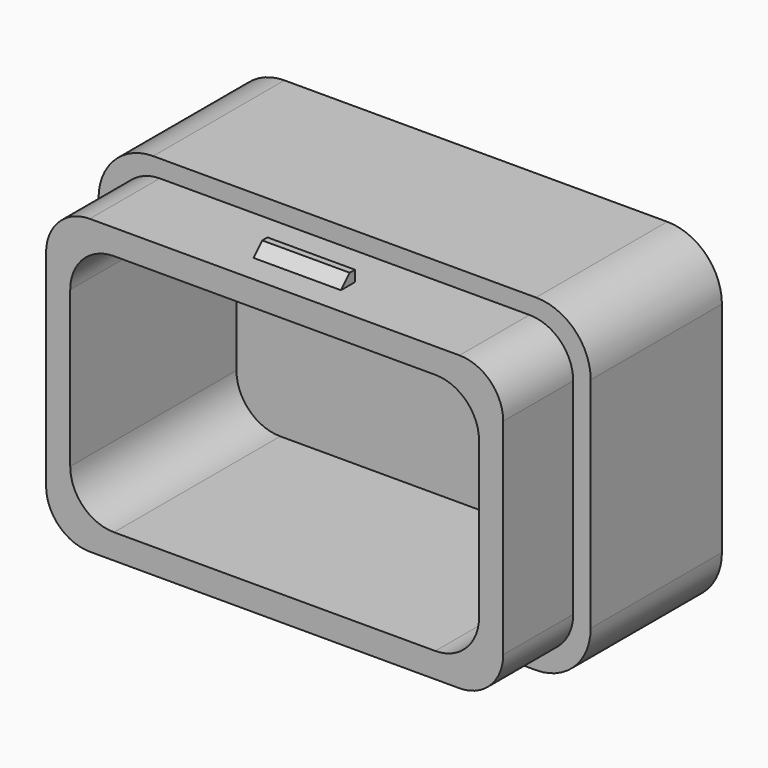
from build123d import *

# Parameters (mm, degrees)
F1_DEPTH = 19.05
F2_DEPTH = 29.21
F3_DEPTH = 5.08
F4_W     = 10.16
F4_H     = 2.032
F5_DEPTH = 1.27
F6_SIZE  = 1.26999


# Not quite as in the source:
# - a fillet or chamfer is up to 0.001 mm smaller than in the source, because OpenCascade refuses the exact size


with BuildPart() as f1:
    # F0 (on Front) → F1 (new body)
    with BuildSketch(Plane.XZ):
        with BuildLine():
            ThreePointArc((28.575, 12.7), (26.7151280605, 17.1901280605), (22.225, 19.05))
            Line((22.225, 19.05), (-22.225, 19.05))
            ThreePointArc((-22.225, 19.05), (-26.7151280605, 17.1901280605), (-28.575, 12.7))
            Line((-28.575, 12.7), (-28.575, -12.7))
            ThreePointArc((-28.575, -12.7), (-26.7151280605, -17.1901280605), (-22.225, -19.05))
            Line((-22.225, -19.05), (22.225, -19.05))
            ThreePointArc((22.225, -19.05), (26.7151280605, -17.1901280605), (28.575, -12.7))
            Line((28.575, -12.7), (28.575, 12.7))
        make_face()
        with BuildLine():
            Line((-21.463, 17.018), (21.463, 17.018))
            ThreePointArc((21.463, 17.018), (25.0551024484, 15.5301024484), (26.543, 11.938))
            Line((26.543, 11.938), (26.543, -11.938))
            ThreePointArc((26.543, -11.938), (25.0551024484, -15.5301024484), (21.463, -17.018))
            Line((21.463, -17.018), (-21.463, -17.018))
            ThreePointArc((-21.463, -17.018), (-25.0551024484, -15.5301024484), (-26.543, -11.938))
            Line((-26.543, -11.938), (-26.543, 11.938))
            ThreePointArc((-26.543, 11.938), (-25.0551024484, 15.5301024484), (-21.463, 17.018))
        make_face(mode=Mode.SUBTRACT)
    extrude(amount=F1_DEPTH)

    # F0 (on Front) → F2 (join)
    with BuildSketch(Plane.XZ):
        with BuildLine():
            ThreePointArc((26.543, 11.938), (25.0551024484, 15.5301024484), (21.463, 17.018))
            Line((21.463, 17.018), (-21.463, 17.018))
            ThreePointArc((-21.463, 17.018), (-25.0551024484, 15.5301024484), (-26.543, 11.938))
            Line((-26.543, 11.938), (-26.543, -11.938))
            ThreePointArc((-26.543, -11.938), (-25.0551024484, -15.5301024484), (-21.463, -17.018))
            Line((-21.463, -17.018), (21.463, -17.018))
            ThreePointArc((21.463, -17.018), (25.0551024484, -15.5301024484), (26.543, -11.938))
            Line((26.543, -11.938), (26.543, 11.938))
        make_face()
        with BuildLine():
            ThreePointArc((-23.7377081066, 9.0361186621), (-22.2498105551, 12.6282211105), (-18.6577081066, 14.1161186621))
            Line((-18.6577081066, 14.1161186621), (18.6577081066, 14.1161186621))
            ThreePointArc((18.6577081066, 14.1161186621), (22.2498105551, 12.6282211105), (23.7377081066, 9.0361186621))
            Line((23.7377081066, 9.0361186621), (23.7377081066, -9.0361186621))
            ThreePointArc((23.7377081066, -9.0361186621), (22.2498105551, -12.6282211105), (18.6577081066, -14.1161186621))
            Line((18.6577081066, -14.1161186621), (-18.6577081066, -14.1161186621))
            ThreePointArc((-18.6577081066, -14.1161186621), (-22.2498105551, -12.6282211105), (-23.7377081066, -9.0361186621))
            Line((-23.7377081066, -9.0361186621), (-23.7377081066, 9.0361186621))
        make_face(mode=Mode.SUBTRACT)
    extrude(amount=F2_DEPTH)

    # F0 (on Front) → F3 (join)
    with BuildSketch(Plane.XZ):
        with BuildLine():
            Line((18.6577081066, 14.1161186621), (-18.6577081066, 14.1161186621))
            ThreePointArc((-18.6577081066, 14.1161186621), (-22.2498105551, 12.6282211105), (-23.7377081066, 9.0361186621))
            Line((-23.7377081066, 9.0361186621), (-23.7377081066, -9.0361186621))
            ThreePointArc((-23.7377081066, -9.0361186621), (-22.2498105551, -12.6282211105), (-18.6577081066, -14.1161186621))
            Line((-18.6577081066, -14.1161186621), (18.6577081066, -14.1161186621))
            ThreePointArc((18.6577081066, -14.1161186621), (22.2498105551, -12.6282211105), (23.7377081066, -9.0361186621))
            Line((23.7377081066, -9.0361186621), (23.7377081066, 9.0361186621))
            ThreePointArc((23.7377081066, 9.0361186621), (22.2498105551, 12.6282211105), (18.6577081066, 14.1161186621))
        make_face()
    extrude(amount=F3_DEPTH)

    # F4 (on face) → F5 (join)
    with BuildSketch(Plane.XY.offset(17.018)):
        with Locations((0, -24.9174)):
            Rectangle(F4_W, F4_H)
    extrude(amount=F5_DEPTH)

    # F6 (size 1.27 in the source; OpenCascade refuses exactly that, so slightly less here)
    f6_edges = [f1.edges().sort_by_distance(p)[0] for p in [
        (0, -25.9334, 18.288),
    ]]
    chamfer(f6_edges, length=F6_SIZE)


solid = f1.part
